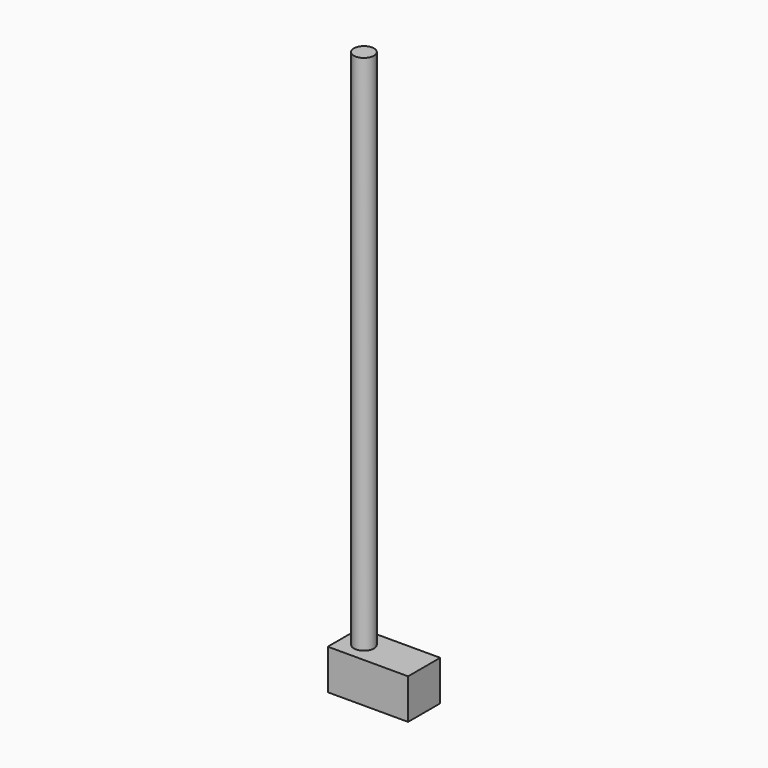
from build123d import *

# Parameters (mm, degrees)
F0_W     = 5.08
F0_H     = 2.54
F1_DEPTH = 2.54
F2_R     = 0.635
F3_DEPTH = 33.02


with BuildPart() as f1:
    # F0 (on Top) → F1 (new body)
    with BuildSketch(Plane.XY):
        with Locations((2.54, -1.27)):
            Rectangle(F0_W, F0_H)
    extrude(amount=F1_DEPTH)

    # F2 (on face) → F3 (join)
    with BuildSketch(Plane.XY.offset(2.54)):
        with Locations((1.27, -1.27)):
            Circle(F2_R)
    extrude(amount=F3_DEPTH)


solid = f1.part
